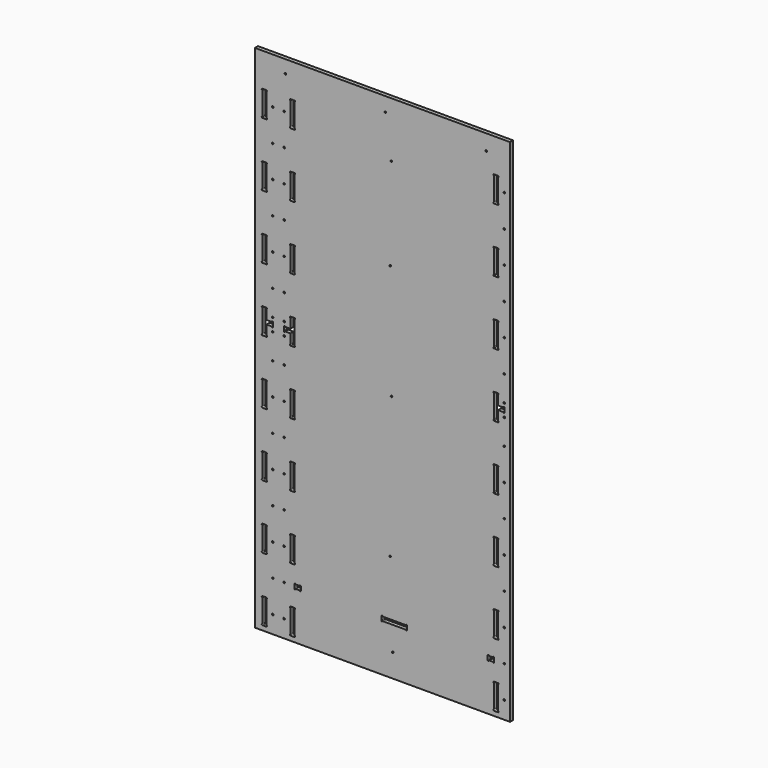
from build123d import *

# Parameters (mm, degrees)
F1_DEPTH = 18


# Not quite as in the source:
# - ends of sketch curves that miss each other by under 0.0002 mm in the source are joined


with BuildPart() as f1:
    # F0 (on Front) → F1 (new body)
    with BuildSketch(Plane.XZ):
        with BuildLine():
            Line((-600, 1063.948034), (-600, -1200))
            Line((-600, -1200), (599.502035, -1200))
            Line((599.502035, -1200), (599.501201, 1063.948272))
            Line((599.501201, 1063.948272), (115.500376, 1063.948245))
            Line((115.500376, 1063.948245), (115.500377, 1053.806799))
            ThreePointArc((115.500377, 1053.806799), (112.3608555537, 1050.5395429438), (108.9803764701, 1053.5568130354))
            Line((108.9803764701, 1053.5568130354), (1.52026, 1053.557046))
            ThreePointArc((1.52026, 1053.557046), (-1.8598651837, 1050.5493557616), (-4.9997393501, 1053.807060001))
            Line((-4.9997393501, 1053.807060001), (-4.999744, 1063.948265))
            Line((-4.999744, 1063.948265), (-600, 1063.948034))
        make_face()
        with BuildLine():
            ThreePointArc((-545.999425, -1057.5382900374), (-542.7418065766, -1060.6737091966), (-545.7494230529, -1064.0496793132))
            Line((-545.7494230529, -1064.0496793132), (-545.749383, -1172.027071))
            ThreePointArc((-545.749383, -1172.027071), (-542.7407774718, -1175.4030773266), (-545.999381, -1178.5384609569))
            Line((-545.999381, -1178.5384609569), (-564.499399, -1178.538468))
            ThreePointArc((-564.499399, -1178.538468), (-567.7570174234, -1175.4030488034), (-564.7494009471, -1172.0270786868))
            Line((-564.7494009471, -1172.0270786868), (-564.749441, -1064.049687))
            ThreePointArc((-564.749441, -1064.049687), (-567.7580465282, -1060.6736806734), (-564.499443, -1057.5382970431))
            Line((-564.499443, -1057.5382970431), (-545.999425, -1057.5382900374))
        make_face(mode=Mode.SUBTRACT)
        with BuildLine():
            ThreePointArc((-516.000128, -1121.775336), (-518.6517784294, -1120.6769864294), (-519.750128, -1118.025336))
            ThreePointArc((-519.750128, -1118.025336), (-518.6517784294, -1115.3736855706), (-516.000128, -1114.275336))
            ThreePointArc((-516.000128, -1114.275336), (-513.3484775706, -1115.3736855706), (-512.250128, -1118.025336))
            ThreePointArc((-512.250128, -1118.025336), (-513.3484775706, -1120.6769864294), (-516.000128, -1121.775336))
        make_face(mode=Mode.SUBTRACT)
        with BuildLine():
            ThreePointArc((-462.491463, -1121.775336), (-465.1431134294, -1120.6769864294), (-466.241463, -1118.025336))
            ThreePointArc((-466.241463, -1118.025336), (-465.1431134294, -1115.3736855706), (-462.491463, -1114.275336))
            ThreePointArc((-462.491463, -1114.275336), (-459.8398125706, -1115.3736855706), (-458.741463, -1118.025336))
            ThreePointArc((-458.741463, -1118.025336), (-459.8398125706, -1120.6769864294), (-462.491463, -1121.775336))
        make_face(mode=Mode.SUBTRACT)
        with BuildLine():
            ThreePointArc((-516.000128, -971.775336), (-518.6517784294, -970.6769864294), (-519.750128, -968.025336))
            ThreePointArc((-519.750128, -968.025336), (-518.6517784294, -965.3736855706), (-516.000128, -964.275336))
            ThreePointArc((-516.000128, -964.275336), (-513.3484775706, -965.3736855706), (-512.250128, -968.025336))
            ThreePointArc((-512.250128, -968.025336), (-513.3484775706, -970.6769864294), (-516.000128, -971.775336))
        make_face(mode=Mode.SUBTRACT)
        with BuildLine():
            ThreePointArc((-462.491463, -971.775336), (-465.1431134294, -970.6769864294), (-466.241463, -968.025336))
            ThreePointArc((-466.241463, -968.025336), (-465.1431134294, -965.3736855706), (-462.491463, -964.275336))
            ThreePointArc((-462.491463, -964.275336), (-459.8398125706, -965.3736855706), (-458.741463, -968.025336))
            ThreePointArc((-458.741463, -968.025336), (-459.8398125706, -970.6769864294), (-462.491463, -971.775336))
        make_face(mode=Mode.SUBTRACT)
        with BuildLine():
            Line((-432.749269, -1172.02703), (-432.749309, -1064.049638))
            ThreePointArc((-432.749309, -1064.049638), (-435.7579145282, -1060.6736316734), (-432.499311, -1057.5382480431))
            Line((-432.499311, -1057.5382480431), (-413.999293, -1057.538241))
            ThreePointArc((-413.999293, -1057.538241), (-410.7416745766, -1060.6736601966), (-413.7492910529, -1064.0496303132))
            Line((-413.7492910529, -1064.0496303132), (-413.749251, -1172.027023))
            ThreePointArc((-413.749251, -1172.027023), (-410.7406454718, -1175.4030293266), (-413.999249, -1178.5384129569))
            Line((-413.999249, -1178.5384129569), (-432.499267, -1178.538419))
            ThreePointArc((-432.499267, -1178.538419), (-435.7568854219, -1175.4029998417), (-432.749269, -1172.02703))
        make_face(mode=Mode.SUBTRACT)
        with BuildLine():
            ThreePointArc((-414.7479649626, -958.781652), (-411.6125458034, -955.5240335766), (-408.2365756868, -958.5316500529))
            Line((-408.2365756868, -958.5316500529), (-390.259321, -958.531643))
            ThreePointArc((-390.259321, -958.531643), (-386.8833146734, -955.5230374718), (-383.7479310431, -958.781641))
            Line((-383.7479310431, -958.781641), (-383.747925, -977.284785))
            ThreePointArc((-383.747925, -977.284785), (-386.8833441966, -980.5424034234), (-390.2593143132, -977.5347869471))
            Line((-390.2593143132, -977.5347869471), (-408.236569, -977.534794))
            ThreePointArc((-408.236569, -977.534794), (-411.6125753266, -980.5433995282), (-414.7479589569, -977.284796))
            Line((-414.7479589569, -977.284796), (-414.7479649626, -958.781652))
        make_face(mode=Mode.SUBTRACT)
        with BuildLine():
            ThreePointArc((-545.999537, -757.5282880373), (-542.7419175958, -760.663706697), (-545.7495340529, -764.0396773132))
            Line((-545.7495340529, -764.0396773132), (-545.749495, -872.016866))
            ThreePointArc((-545.749495, -872.016866), (-542.7408894527, -875.3928718269), (-545.999492, -878.5282559571))
            Line((-545.999492, -878.5282559571), (-564.49951, -878.528262))
            ThreePointArc((-564.49951, -878.528262), (-567.7571294027, -875.3928433414), (-564.7495130237, -872.0168726927))
            Line((-564.7495130237, -872.0168726927), (-564.749552, -764.039685))
            ThreePointArc((-564.749552, -764.039685), (-567.7581575473, -760.6636791731), (-564.499555, -757.5282950429))
            Line((-564.499555, -757.5282950429), (-545.999537, -757.5282880373))
        make_face(mode=Mode.SUBTRACT)
        with BuildLine():
            ThreePointArc((-516.000128, -821.775336), (-518.6517784294, -820.6769864294), (-519.750128, -818.025336))
            ThreePointArc((-519.750128, -818.025336), (-518.6517784294, -815.3736855706), (-516.000128, -814.275336))
            ThreePointArc((-516.000128, -814.275336), (-513.3484775706, -815.3736855706), (-512.250128, -818.025336))
            ThreePointArc((-512.250128, -818.025336), (-513.3484775706, -820.6769864294), (-516.000128, -821.775336))
        make_face(mode=Mode.SUBTRACT)
        with BuildLine():
            ThreePointArc((-462.491463, -821.775336), (-465.1431134294, -820.6769864294), (-466.241463, -818.025336))
            ThreePointArc((-466.241463, -818.025336), (-465.1431134294, -815.3736855706), (-462.491463, -814.275336))
            ThreePointArc((-462.491463, -814.275336), (-459.8398125706, -815.3736855706), (-458.741463, -818.025336))
            ThreePointArc((-458.741463, -818.025336), (-459.8398125706, -820.6769864294), (-462.491463, -821.775336))
        make_face(mode=Mode.SUBTRACT)
        with BuildLine():
            ThreePointArc((-516.000128, -671.775336), (-518.6517784294, -670.6769864294), (-519.750128, -668.025336))
            ThreePointArc((-519.750128, -668.025336), (-518.6517784294, -665.3736855706), (-516.000128, -664.275336))
            ThreePointArc((-516.000128, -664.275336), (-513.3484775706, -665.3736855706), (-512.250128, -668.025336))
            ThreePointArc((-512.250128, -668.025336), (-513.3484775706, -670.6769864294), (-516.000128, -671.775336))
        make_face(mode=Mode.SUBTRACT)
        with BuildLine():
            ThreePointArc((-462.491463, -671.775336), (-465.1431134294, -670.6769864294), (-466.241463, -668.025336))
            ThreePointArc((-466.241463, -668.025336), (-465.1431134294, -665.3736855706), (-462.491463, -664.275336))
            ThreePointArc((-462.491463, -664.275336), (-459.8398125706, -665.3736855706), (-458.741463, -668.025336))
            ThreePointArc((-458.741463, -668.025336), (-459.8398125706, -670.6769864294), (-462.491463, -671.775336))
        make_face(mode=Mode.SUBTRACT)
        with BuildLine():
            ThreePointArc((-432.7494189421, -764.0396352449), (-435.7580235481, -760.6636302113), (-432.499422, -757.5282470429))
            Line((-432.499422, -757.5282470429), (-413.999404, -757.52824))
            ThreePointArc((-413.999404, -757.52824), (-410.7417845973, -760.6636586586), (-413.7494009763, -764.0396293073))
            Line((-413.7494009763, -764.0396293073), (-413.749363, -872.016817))
            ThreePointArc((-413.749363, -872.016817), (-410.7407574527, -875.3928228269), (-413.99936, -878.5282069571))
            Line((-413.99936, -878.5282069571), (-432.499377, -878.528214))
            ThreePointArc((-432.499377, -878.528214), (-435.7569964042, -875.392795303), (-432.7493799471, -872.0168246868))
            Line((-432.7493799471, -872.0168246868), (-432.7494189421, -764.0396352449))
        make_face(mode=Mode.SUBTRACT)
        with BuildLine():
            ThreePointArc((-545.999646, -457.5277780374), (-542.7420275766, -460.6631971966), (-545.7496440529, -464.0391673132))
            Line((-545.7496440529, -464.0391673132), (-545.749604, -572.01656))
            ThreePointArc((-545.749604, -572.01656), (-542.7409984718, -575.3925663266), (-545.999602, -578.5279499569))
            Line((-545.999602, -578.5279499569), (-564.49962, -578.527957))
            ThreePointArc((-564.49962, -578.527957), (-567.7572384234, -575.3925378034), (-564.7496219471, -572.0165676868))
            Line((-564.7496219471, -572.0165676868), (-564.749662, -464.039175))
            ThreePointArc((-564.749662, -464.039175), (-567.7582675282, -460.6631686734), (-564.499664, -457.5277850431))
            Line((-564.499664, -457.5277850431), (-545.999646, -457.5277780374))
        make_face(mode=Mode.SUBTRACT)
        with BuildLine():
            ThreePointArc((-516.000128, -521.775336), (-518.6517784294, -520.6769864294), (-519.750128, -518.025336))
            ThreePointArc((-519.750128, -518.025336), (-518.6517784294, -515.3736855706), (-516.000128, -514.275336))
            ThreePointArc((-516.000128, -514.275336), (-513.3484775706, -515.3736855706), (-512.250128, -518.025336))
            ThreePointArc((-512.250128, -518.025336), (-513.3484775706, -520.6769864294), (-516.000128, -521.775336))
        make_face(mode=Mode.SUBTRACT)
        with BuildLine():
            ThreePointArc((-462.491463, -521.775336), (-465.1431134294, -520.6769864294), (-466.241463, -518.025336))
            ThreePointArc((-466.241463, -518.025336), (-465.1431134294, -515.3736855706), (-462.491463, -514.275336))
            ThreePointArc((-462.491463, -514.275336), (-459.8398125706, -515.3736855706), (-458.741463, -518.025336))
            ThreePointArc((-458.741463, -518.025336), (-459.8398125706, -520.6769864294), (-462.491463, -521.775336))
        make_face(mode=Mode.SUBTRACT)
        with BuildLine():
            ThreePointArc((-516.000128, -371.775336), (-518.6517784294, -370.6769864294), (-519.750128, -368.025336))
            ThreePointArc((-519.750128, -368.025336), (-518.6517784294, -365.3736855706), (-516.000128, -364.275336))
            ThreePointArc((-516.000128, -364.275336), (-513.3484775706, -365.3736855706), (-512.250128, -368.025336))
            ThreePointArc((-512.250128, -368.025336), (-513.3484775706, -370.6769864294), (-516.000128, -371.775336))
        make_face(mode=Mode.SUBTRACT)
        with BuildLine():
            ThreePointArc((-462.491463, -371.775336), (-465.1431134294, -370.6769864294), (-466.241463, -368.025336))
            ThreePointArc((-466.241463, -368.025336), (-465.1431134294, -365.3736855706), (-462.491463, -364.275336))
            ThreePointArc((-462.491463, -364.275336), (-459.8398125706, -365.3736855706), (-458.741463, -368.025336))
            ThreePointArc((-458.741463, -368.025336), (-459.8398125706, -370.6769864294), (-462.491463, -371.775336))
        make_face(mode=Mode.SUBTRACT)
        with BuildLine():
            ThreePointArc((-432.7495300186, -464.039126242), (-435.7581355282, -460.6631196734), (-432.499532, -457.5277360431))
            Line((-432.499532, -457.5277360431), (-413.999514, -457.52773))
            ThreePointArc((-413.999514, -457.52773), (-410.7418955781, -460.6631491583), (-413.7495119763, -464.0391193073))
            Line((-413.7495119763, -464.0391193073), (-413.749473, -572.016307))
            ThreePointArc((-413.749473, -572.016307), (-410.7408674718, -575.3923133266), (-413.999471, -578.5276969569))
            Line((-413.999471, -578.5276969569), (-432.499488, -578.527704))
            ThreePointArc((-432.499488, -578.527704), (-435.7571064234, -575.3922848034), (-432.7494899471, -572.0163146868))
            Line((-432.7494899471, -572.0163146868), (-432.7495300186, -464.039126242))
        make_face(mode=Mode.SUBTRACT)
        with BuildLine():
            ThreePointArc((-545.999757, -157.5272680374), (-542.7421385766, -160.6626871966), (-545.7497550529, -164.0386573132))
            Line((-545.7497550529, -164.0386573132), (-545.749715, -272.01605))
            ThreePointArc((-545.749715, -272.01605), (-542.7411094527, -275.3920558269), (-545.999712, -278.5274399571))
            Line((-545.999712, -278.5274399571), (-564.49973, -278.527446))
            ThreePointArc((-564.49973, -278.527446), (-567.7573494027, -275.3920273414), (-564.7497330237, -272.0160566927))
            Line((-564.7497330237, -272.0160566927), (-564.749773, -164.038665))
            ThreePointArc((-564.749773, -164.038665), (-567.7583785282, -160.6626586734), (-564.499775, -157.5272750431))
            Line((-564.499775, -157.5272750431), (-545.999757, -157.5272680374))
        make_face(mode=Mode.SUBTRACT)
        with BuildLine():
            ThreePointArc((-516.000128, -221.775336), (-518.6517784294, -220.6769864294), (-519.750128, -218.025336))
            ThreePointArc((-519.750128, -218.025336), (-518.6517784294, -215.3736855706), (-516.000128, -214.275336))
            ThreePointArc((-516.000128, -214.275336), (-513.3484775706, -215.3736855706), (-512.250128, -218.025336))
            ThreePointArc((-512.250128, -218.025336), (-513.3484775706, -220.6769864294), (-516.000128, -221.775336))
        make_face(mode=Mode.SUBTRACT)
        with BuildLine():
            ThreePointArc((-462.491463, -221.775336), (-465.1431134294, -220.6769864294), (-466.241463, -218.025336))
            ThreePointArc((-466.241463, -218.025336), (-465.1431134294, -215.3736855706), (-462.491463, -214.275336))
            ThreePointArc((-462.491463, -214.275336), (-459.8398125706, -215.3736855706), (-458.741463, -218.025336))
            ThreePointArc((-458.741463, -218.025336), (-459.8398125706, -220.6769864294), (-462.491463, -221.775336))
        make_face(mode=Mode.SUBTRACT)
        with BuildLine():
            ThreePointArc((-516.000128, -71.775336), (-518.6517784294, -70.6769864294), (-519.750128, -68.025336))
            ThreePointArc((-519.750128, -68.025336), (-518.6517784294, -65.3736855706), (-516.000128, -64.275336))
            ThreePointArc((-516.000128, -64.275336), (-513.3484775706, -65.3736855706), (-512.250128, -68.025336))
            ThreePointArc((-512.250128, -68.025336), (-513.3484775706, -70.6769864294), (-516.000128, -71.775336))
        make_face(mode=Mode.SUBTRACT)
        with BuildLine():
            ThreePointArc((-462.491463, -71.775336), (-465.1431134294, -70.6769864294), (-466.241463, -68.025336))
            ThreePointArc((-466.241463, -68.025336), (-465.1431134294, -65.3736855706), (-462.491463, -64.275336))
            ThreePointArc((-462.491463, -64.275336), (-459.8398125706, -65.3736855706), (-458.741463, -68.025336))
            ThreePointArc((-458.741463, -68.025336), (-459.8398125706, -70.6769864294), (-462.491463, -71.775336))
        make_face(mode=Mode.SUBTRACT)
        with BuildLine():
            ThreePointArc((-432.7496410186, -164.038616242), (-435.7582465282, -160.6626096734), (-432.499643, -157.5272260431))
            Line((-432.499643, -157.5272260431), (-413.999625, -157.527219))
            ThreePointArc((-413.999625, -157.527219), (-410.7420065766, -160.6626381966), (-413.7496230529, -164.0386083132))
            Line((-413.7496230529, -164.0386083132), (-413.749584, -272.015797))
            ThreePointArc((-413.749584, -272.015797), (-410.7409784527, -275.3918028269), (-413.999581, -278.5271869571))
            Line((-413.999581, -278.5271869571), (-432.499598, -278.527193))
            ThreePointArc((-432.499598, -278.527193), (-435.7572174027, -275.3917743414), (-432.7496010237, -272.0158036927))
            Line((-432.7496010237, -272.0158036927), (-432.7496410186, -164.038616242))
        make_face(mode=Mode.SUBTRACT)
        with BuildLine():
            ThreePointArc((44.445, -1090.918442), (45.5433495706, -1088.2667915706), (48.195, -1087.168442))
            ThreePointArc((48.195, -1087.168442), (50.8466504294, -1088.2667915706), (51.945, -1090.918442))
            ThreePointArc((51.945, -1090.918442), (50.8466504294, -1093.5700924294), (48.195, -1094.668442))
            ThreePointArc((48.195, -1094.668442), (45.5433495706, -1093.5700924294), (44.445, -1090.918442))
        make_face(mode=Mode.SUBTRACT)
        with BuildLine():
            ThreePointArc((1.263840242, -977.5348170186), (-2.1121658269, -980.5434225473), (-5.2475499571, -977.28482))
            Line((-5.2475499571, -977.28482), (-5.247556, -958.781327))
            ThreePointArc((-5.247556, -958.781327), (-2.1121368034, -955.5237085766), (1.2638333132, -958.5313250529))
            Line((1.2638333132, -958.5313250529), (109.241178, -958.531285))
            ThreePointArc((109.241178, -958.531285), (112.6171843266, -955.5226794718), (115.7525679569, -958.781283))
            Line((115.7525679569, -958.781283), (115.752574, -977.284775))
            ThreePointArc((115.752574, -977.284775), (112.6171548034, -980.5423934234), (109.2411846868, -977.5347769471))
            Line((109.2411846868, -977.5347769471), (1.263840242, -977.5348170186))
        make_face(mode=Mode.SUBTRACT)
        with BuildLine():
            ThreePointArc((32.71, -697.766442), (33.8083495706, -695.1147915706), (36.46, -694.016442))
            ThreePointArc((36.46, -694.016442), (39.1116504294, -695.1147915706), (40.21, -697.766442))
            ThreePointArc((40.21, -697.766442), (39.1116504294, -700.4180924294), (36.46, -701.516442))
            ThreePointArc((36.46, -701.516442), (33.8083495706, -700.4180924294), (32.71, -697.766442))
        make_face(mode=Mode.SUBTRACT)
        with BuildLine():
            ThreePointArc((524.2514499814, -1064.044670242), (521.2428444527, -1060.6686641731), (524.501447, -1057.5332800429))
            Line((524.501447, -1057.5332800429), (543.001465, -1057.533274))
            ThreePointArc((543.001465, -1057.533274), (546.2590844027, -1060.6686926586), (543.2514680237, -1064.0446633073))
            Line((543.2514680237, -1064.0446633073), (543.251507, -1172.022004))
            ThreePointArc((543.251507, -1172.022004), (546.2601125473, -1175.3980098269), (543.00151, -1178.5333939571))
            Line((543.00151, -1178.5333939571), (524.501492, -1178.5334))
            ThreePointArc((524.501492, -1178.5334), (521.2438725973, -1175.3979813414), (524.2514889763, -1172.0220106927))
            Line((524.2514889763, -1172.0220106927), (524.2514499814, -1064.044670242))
        make_face(mode=Mode.SUBTRACT)
        with BuildLine():
            ThreePointArc((572.885133, -1121.775336), (570.2334825706, -1120.6769864294), (569.135133, -1118.025336))
            ThreePointArc((569.135133, -1118.025336), (570.2334825706, -1115.3736855706), (572.885133, -1114.275336))
            ThreePointArc((572.885133, -1114.275336), (575.5367834294, -1115.3736855706), (576.635133, -1118.025336))
            ThreePointArc((576.635133, -1118.025336), (575.5367834294, -1120.6769864294), (572.885133, -1121.775336))
        make_face(mode=Mode.SUBTRACT)
        with BuildLine():
            ThreePointArc((500.7643391657, -977.5348480127), (497.3883316756, -980.5434524898), (494.2529490432, -977.284848))
            Line((494.2529490432, -977.284848), (494.252943, -958.78093))
            ThreePointArc((494.252943, -958.78093), (497.3883606992, -955.5233096341), (500.7643322366, -958.5309250588))
            Line((500.7643322366, -958.5309250588), (518.741583, -958.530911))
            ThreePointArc((518.741583, -958.530911), (522.1175878291, -955.5223044144), (525.2529729572, -958.780906))
            Line((525.2529729572, -958.780906), (525.252979, -977.28485))
            ThreePointArc((525.252979, -977.28485), (522.1175583074, -980.5424674808), (518.7415895336, -977.5348489589))
            Line((518.7415895336, -977.5348489589), (500.7643391657, -977.5348480127))
        make_face(mode=Mode.SUBTRACT)
        with BuildLine():
            ThreePointArc((572.885133, -971.775336), (570.2334825706, -970.6769864294), (569.135133, -968.025336))
            ThreePointArc((569.135133, -968.025336), (570.2334825706, -965.3736855706), (572.885133, -964.275336))
            ThreePointArc((572.885133, -964.275336), (575.5367834294, -965.3736855706), (576.635133, -968.025336))
            ThreePointArc((576.635133, -968.025336), (575.5367834294, -970.6769864294), (572.885133, -971.775336))
        make_face(mode=Mode.SUBTRACT)
        with BuildLine():
            ThreePointArc((543.2513960186, -872.021078758), (546.2600015282, -875.3970853266), (543.001398, -878.5324689569))
            Line((543.001398, -878.5324689569), (524.501381, -878.532476))
            ThreePointArc((524.501381, -878.532476), (521.2437625766, -875.3970568034), (524.2513790529, -872.0210866868))
            Line((524.2513790529, -872.0210866868), (524.251338, -764.04395))
            ThreePointArc((524.251338, -764.04395), (521.2427324527, -760.6679441731), (524.501335, -757.5325600429))
            Line((524.501335, -757.5325600429), (543.001353, -757.532553))
            ThreePointArc((543.001353, -757.532553), (546.2589724042, -760.667971697), (543.2513559471, -764.0439423132))
            Line((543.2513559471, -764.0439423132), (543.2513960186, -872.021078758))
        make_face(mode=Mode.SUBTRACT)
        with BuildLine():
            ThreePointArc((572.885133, -821.775336), (570.2334825706, -820.6769864294), (569.135133, -818.025336))
            ThreePointArc((569.135133, -818.025336), (570.2334825706, -815.3736855706), (572.885133, -814.275336))
            ThreePointArc((572.885133, -814.275336), (575.5367834294, -815.3736855706), (576.635133, -818.025336))
            ThreePointArc((576.635133, -818.025336), (575.5367834294, -820.6769864294), (572.885133, -821.775336))
        make_face(mode=Mode.SUBTRACT)
        with BuildLine():
            ThreePointArc((572.885133, -671.775336), (570.2334825706, -670.6769864294), (569.135133, -668.025336))
            ThreePointArc((569.135133, -668.025336), (570.2334825706, -665.3736855706), (572.885133, -664.275336))
            ThreePointArc((572.885133, -664.275336), (575.5367834294, -665.3736855706), (576.635133, -668.025336))
            ThreePointArc((576.635133, -668.025336), (575.5367834294, -670.6769864294), (572.885133, -671.775336))
        make_face(mode=Mode.SUBTRACT)
        with BuildLine():
            ThreePointArc((38.577, -33.984585), (39.6753495706, -31.3329345706), (42.327, -30.234585))
            ThreePointArc((42.327, -30.234585), (44.9786504294, -31.3329345706), (46.077, -33.984585))
            ThreePointArc((46.077, -33.984585), (44.9786504294, -36.6362354294), (42.327, -37.734585))
            ThreePointArc((42.327, -37.734585), (39.6753495706, -36.6362354294), (38.577, -33.984585))
        make_face(mode=Mode.SUBTRACT)
        with BuildLine():
            ThreePointArc((524.501271, -578.5319659627), (521.2436515958, -575.396547303), (524.2512680529, -572.0205766868))
            Line((524.2512680529, -572.0205766868), (524.251227, -464.04344))
            ThreePointArc((524.251227, -464.04344), (521.2426214718, -460.6674336734), (524.501225, -457.5320500431))
            Line((524.501225, -457.5320500431), (543.001243, -457.532043))
            ThreePointArc((543.001243, -457.532043), (546.2588614234, -460.6674621966), (543.2512449471, -464.0434323132))
            Line((543.2512449471, -464.0434323132), (543.251285, -572.020569))
            ThreePointArc((543.251285, -572.020569), (546.2598905282, -575.3965753266), (543.001287, -578.5319589569))
            Line((543.001287, -578.5319589569), (524.501271, -578.5319659627))
        make_face(mode=Mode.SUBTRACT)
        with BuildLine():
            ThreePointArc((572.885133, -521.775336), (570.2334825706, -520.6769864294), (569.135133, -518.025336))
            ThreePointArc((569.135133, -518.025336), (570.2334825706, -515.3736855706), (572.885133, -514.275336))
            ThreePointArc((572.885133, -514.275336), (575.5367834294, -515.3736855706), (576.635133, -518.025336))
            ThreePointArc((576.635133, -518.025336), (575.5367834294, -520.6769864294), (572.885133, -521.775336))
        make_face(mode=Mode.SUBTRACT)
        with BuildLine():
            ThreePointArc((572.885133, -371.775336), (570.2334825706, -370.6769864294), (569.135133, -368.025336))
            ThreePointArc((569.135133, -368.025336), (570.2334825706, -365.3736855706), (572.885133, -364.275336))
            ThreePointArc((572.885133, -364.275336), (575.5367834294, -365.3736855706), (576.635133, -368.025336))
            ThreePointArc((576.635133, -368.025336), (575.5367834294, -370.6769864294), (572.885133, -371.775336))
        make_face(mode=Mode.SUBTRACT)
        with BuildLine():
            ThreePointArc((543.2511740186, -272.020058758), (546.2597795473, -275.3960648269), (543.001177, -278.5314489571))
            Line((543.001177, -278.5314489571), (524.50116, -278.531455))
            ThreePointArc((524.50116, -278.531455), (521.2435415781, -275.3960358417), (524.2511579763, -272.0200656927))
            Line((524.2511579763, -272.0200656927), (524.251117, -164.04293))
            ThreePointArc((524.251117, -164.04293), (521.2425114527, -160.6669241731), (524.501114, -157.5315400429))
            Line((524.501114, -157.5315400429), (543.001132, -157.531533))
            ThreePointArc((543.001132, -157.531533), (546.2587514042, -160.666951697), (543.2511349471, -164.0429223132))
            Line((543.2511349471, -164.0429223132), (543.2511740186, -272.020058758))
        make_face(mode=Mode.SUBTRACT)
        with BuildLine():
            ThreePointArc((572.885133, -221.775336), (570.2334825706, -220.6769864294), (569.135133, -218.025336))
            ThreePointArc((569.135133, -218.025336), (570.2334825706, -215.3736855706), (572.885133, -214.275336))
            ThreePointArc((572.885133, -214.275336), (575.5367834294, -215.3736855706), (576.635133, -218.025336))
            ThreePointArc((576.635133, -218.025336), (575.5367834294, -220.6769864294), (572.885133, -221.775336))
        make_face(mode=Mode.SUBTRACT)
        with BuildLine():
            ThreePointArc((572.885133, -71.775336), (570.2334825706, -70.6769864294), (569.135133, -68.025336))
            ThreePointArc((569.135133, -68.025336), (570.2334825706, -65.3736855706), (572.885133, -64.275336))
            ThreePointArc((572.885133, -64.275336), (575.5367834294, -65.3736855706), (576.635133, -68.025336))
            ThreePointArc((576.635133, -68.025336), (575.5367834294, -70.6769864294), (572.885133, -71.775336))
        make_face(mode=Mode.SUBTRACT)
        with BuildLine():
            ThreePointArc((-545.999868, 142.4669129627), (-542.7422485958, 139.331494303), (-545.7498650529, 135.9555236868))
            Line((-545.7498650529, 135.9555236868), (-545.749849, 91.466836))
            Line((-545.749849, 91.466836), (-521.261208, 91.466846))
            ThreePointArc((-521.261208, 91.466846), (-517.8852016734, 94.4754515282), (-514.7498180431, 91.216848))
            Line((-514.7498180431, 91.216848), (-514.749811, 72.716827))
            ThreePointArc((-514.749811, 72.716827), (-517.8852521863, 69.4592297324), (-521.2612020042, 72.4668689997))
            Line((-521.2612020042, 72.4668689997), (-545.749843, 72.467028))
            Line((-545.749843, 72.467028), (-545.749827, 27.978336))
            ThreePointArc((-545.749827, 27.978336), (-542.7412214527, 24.6023301731), (-545.999824, 21.4669460429))
            Line((-545.999824, 21.4669460429), (-564.499841, 21.466939))
            ThreePointArc((-564.499841, 21.466939), (-567.7574594234, 24.6023581966), (-564.7498429471, 27.9783283132))
            Line((-564.7498429471, 27.9783283132), (-564.749884, 135.955516))
            ThreePointArc((-564.749884, 135.955516), (-567.7584895473, 139.3315218269), (-564.499887, 142.4669059571))
            Line((-564.499887, 142.4669059571), (-545.999868, 142.4669129627))
        make_face(mode=Mode.SUBTRACT)
        with BuildLine():
            ThreePointArc((-516.000128, 48.224664), (-518.6517784294, 49.3230135706), (-519.750128, 51.974664))
            ThreePointArc((-519.750128, 51.974664), (-518.6517784294, 54.6263144294), (-516.000128, 55.724664))
            ThreePointArc((-516.000128, 55.724664), (-513.3484775706, 54.6263144294), (-512.250128, 51.974664))
            ThreePointArc((-512.250128, 51.974664), (-513.3484775706, 49.3230135706), (-516.000128, 48.224664))
        make_face(mode=Mode.SUBTRACT)
        with BuildLine():
            ThreePointArc((-462.491463, 48.224664), (-465.1431134294, 49.3230135706), (-466.241463, 51.974664))
            ThreePointArc((-466.241463, 51.974664), (-465.1431134294, 54.6263144294), (-462.491463, 55.724664))
            ThreePointArc((-462.491463, 55.724664), (-459.8398125706, 54.6263144294), (-458.741463, 51.974664))
            ThreePointArc((-458.741463, 51.974664), (-459.8398125706, 49.3230135706), (-462.491463, 48.224664))
        make_face(mode=Mode.SUBTRACT)
        with BuildLine():
            ThreePointArc((-516.000128, 108.224664), (-518.6517784294, 109.3230135706), (-519.750128, 111.974664))
            ThreePointArc((-519.750128, 111.974664), (-518.6517784294, 114.6263144294), (-516.000128, 115.724664))
            ThreePointArc((-516.000128, 115.724664), (-513.3484775706, 114.6263144294), (-512.250128, 111.974664))
            ThreePointArc((-512.250128, 111.974664), (-513.3484775706, 109.3230135706), (-516.000128, 108.224664))
        make_face(mode=Mode.SUBTRACT)
        with BuildLine():
            ThreePointArc((-462.491463, 108.224664), (-465.1431134294, 109.3230135706), (-466.241463, 111.974664))
            ThreePointArc((-466.241463, 111.974664), (-465.1431134294, 114.6263144294), (-462.491463, 115.724664))
            ThreePointArc((-462.491463, 115.724664), (-459.8398125706, 114.6263144294), (-458.741463, 111.974664))
            ThreePointArc((-458.741463, 111.974664), (-459.8398125706, 109.3230135706), (-462.491463, 108.224664))
        make_face(mode=Mode.SUBTRACT)
        with BuildLine():
            ThreePointArc((-516.000128, 228.224664), (-518.6517784294, 229.3230135706), (-519.750128, 231.974664))
            ThreePointArc((-519.750128, 231.974664), (-518.6517784294, 234.6263144294), (-516.000128, 235.724664))
            ThreePointArc((-516.000128, 235.724664), (-513.3484775706, 234.6263144294), (-512.250128, 231.974664))
            ThreePointArc((-512.250128, 231.974664), (-513.3484775706, 229.3230135706), (-516.000128, 228.224664))
        make_face(mode=Mode.SUBTRACT)
        with BuildLine():
            ThreePointArc((-462.491463, 228.224664), (-465.1431134294, 229.3230135706), (-466.241463, 231.974664))
            ThreePointArc((-466.241463, 231.974664), (-465.1431134294, 234.6263144294), (-462.491463, 235.724664))
            ThreePointArc((-462.491463, 235.724664), (-459.8398125706, 234.6263144294), (-458.741463, 231.974664))
            ThreePointArc((-458.741463, 231.974664), (-459.8398125706, 229.3230135706), (-462.491463, 228.224664))
        make_face(mode=Mode.SUBTRACT)
        with BuildLine():
            ThreePointArc((-432.7497510186, 135.955564758), (-435.7583565473, 139.3315708269), (-432.499754, 142.4669549571))
            Line((-432.499754, 142.4669549571), (-413.999736, 142.466962))
            ThreePointArc((-413.999736, 142.466962), (-410.7421165958, 139.331543303), (-413.7497330529, 135.9555726868))
            Line((-413.7497330529, 135.9555726868), (-413.749694, 27.978385))
            ThreePointArc((-413.749694, 27.978385), (-410.7410884718, 24.6023786734), (-413.999692, 21.4669950431))
            Line((-413.999692, 21.4669950431), (-432.499709, 21.466988))
            ThreePointArc((-432.499709, 21.466988), (-435.7573274234, 24.6024071966), (-432.7497109471, 27.9783773132))
            Line((-432.7497109471, 27.9783773132), (-432.749728, 72.46686))
            Line((-432.749728, 72.46686), (-457.238369, 72.466851))
            ThreePointArc((-457.238369, 72.466851), (-460.6143753266, 69.4582454718), (-463.7497589569, 72.716849))
            Line((-463.7497589569, 72.716849), (-463.749766, 91.216864))
            ThreePointArc((-463.749766, 91.216864), (-460.6143688314, 94.4745035776), (-457.2383783839, 91.4669099704))
            Line((-457.2383783839, 91.4669099704), (-432.749736, 91.467088))
            Line((-432.749736, 91.467088), (-432.7497510186, 135.955564758))
        make_face(mode=Mode.SUBTRACT)
        with BuildLine():
            ThreePointArc((-545.999978, 442.4735929626), (-542.7423595766, 439.3381738034), (-545.7499760529, 435.9622036868))
            Line((-545.7499760529, 435.9622036868), (-545.749936, 327.984812))
            ThreePointArc((-545.749936, 327.984812), (-542.7413304718, 324.6088056734), (-545.999934, 321.4734220431))
            Line((-545.999934, 321.4734220431), (-564.499952, 321.473415))
            ThreePointArc((-564.499952, 321.473415), (-567.7575704234, 324.6088341966), (-564.7499539471, 327.9848043132))
            Line((-564.7499539471, 327.9848043132), (-564.749994, 435.962196))
            ThreePointArc((-564.749994, 435.962196), (-567.7585995282, 439.3382023266), (-564.499996, 442.4735859569))
            Line((-564.499996, 442.4735859569), (-545.999978, 442.4735929626))
        make_face(mode=Mode.SUBTRACT)
        with BuildLine():
            ThreePointArc((-516.000128, 378.224664), (-518.6517784294, 379.3230135706), (-519.750128, 381.974664))
            ThreePointArc((-519.750128, 381.974664), (-518.6517784294, 384.6263144294), (-516.000128, 385.724664))
            ThreePointArc((-516.000128, 385.724664), (-513.3484775706, 384.6263144294), (-512.250128, 381.974664))
            ThreePointArc((-512.250128, 381.974664), (-513.3484775706, 379.3230135706), (-516.000128, 378.224664))
        make_face(mode=Mode.SUBTRACT)
        with BuildLine():
            ThreePointArc((-462.491463, 378.224664), (-465.1431134294, 379.3230135706), (-466.241463, 381.974664))
            ThreePointArc((-466.241463, 381.974664), (-465.1431134294, 384.6263144294), (-462.491463, 385.724664))
            ThreePointArc((-462.491463, 385.724664), (-459.8398125706, 384.6263144294), (-458.741463, 381.974664))
            ThreePointArc((-458.741463, 381.974664), (-459.8398125706, 379.3230135706), (-462.491463, 378.224664))
        make_face(mode=Mode.SUBTRACT)
        with BuildLine():
            ThreePointArc((-516.000128, 528.224664), (-518.6517784294, 529.3230135706), (-519.750128, 531.974664))
            ThreePointArc((-519.750128, 531.974664), (-518.6517784294, 534.6263144294), (-516.000128, 535.724664))
            ThreePointArc((-516.000128, 535.724664), (-513.3484775706, 534.6263144294), (-512.250128, 531.974664))
            ThreePointArc((-512.250128, 531.974664), (-513.3484775706, 529.3230135706), (-516.000128, 528.224664))
        make_face(mode=Mode.SUBTRACT)
        with BuildLine():
            ThreePointArc((-462.491463, 528.224664), (-465.1431134294, 529.3230135706), (-466.241463, 531.974664))
            ThreePointArc((-466.241463, 531.974664), (-465.1431134294, 534.6263144294), (-462.491463, 535.724664))
            ThreePointArc((-462.491463, 535.724664), (-459.8398125706, 534.6263144294), (-458.741463, 531.974664))
            ThreePointArc((-458.741463, 531.974664), (-459.8398125706, 529.3230135706), (-462.491463, 528.224664))
        make_face(mode=Mode.SUBTRACT)
        with BuildLine():
            ThreePointArc((-432.7498620186, 435.962244758), (-435.7584675282, 439.3382513266), (-432.499864, 442.4736349569))
            Line((-432.499864, 442.4736349569), (-413.999846, 442.473642))
            ThreePointArc((-413.999846, 442.473642), (-410.7422275766, 439.3382228034), (-413.7498440529, 435.9622526868))
            Line((-413.7498440529, 435.9622526868), (-413.749805, 327.985065))
            ThreePointArc((-413.749805, 327.985065), (-410.7411994718, 324.6090586734), (-413.999803, 321.4736750431))
            Line((-413.999803, 321.4736750431), (-432.49982, 321.473668))
            ThreePointArc((-432.49982, 321.473668), (-435.7574384234, 324.6090871966), (-432.7498219471, 327.9850573132))
            Line((-432.7498219471, 327.9850573132), (-432.7498620186, 435.962244758))
        make_face(mode=Mode.SUBTRACT)
        Polygon((-32.274155, 136.734384), (-49.831488, 136.734384), (-49.831488, 156.705051), (-32.274155, 156.705051), (-31.779779, 156.701647), (-31.288275, 156.672696), (-30.800575, 156.61859), (-30.317613, 156.539717), (-29.840323, 156.43647), (-29.369639, 156.309238), (-28.906494, 156.158413), (-28.451821, 155.984384), (-28.006555, 155.787543), (-27.571629, 155.56828), (-27.147976, 155.326985), (-26.73653, 155.064051), (-26.338224, 154.779866), (-25.953993, 154.474821), (-25.58477, 154.149308), (-25.231488, 153.803717), (-24.891049, 153.452209), (-24.569978, 153.08528), (-24.26864, 152.703819), (-23.987405, 152.308717), (-23.726638, 151.900866), (-23.486707, 151.481155), (-23.267979, 151.050475), (-23.070821, 150.609717), (-22.895601, 150.159772), (-22.742686, 149.70153), (-22.612443, 149.235881), (-22.505238, 148.763717), (-22.42144, 148.285928), (-22.361415, 147.803405), (-22.325531, 147.317038), (-22.314155, 146.827717), (-22.311185, 146.326156), (-22.334025, 145.827103), (-22.382293, 145.331502), (-22.455613, 144.840301), (-22.553605, 144.354442), (-22.675889, 143.874873), (-22.822088, 143.402539), (-22.991821, 142.938384), (-23.184711, 142.483354), (-23.400379, 142.038394), (-23.638444, 141.60445), (-23.89853, 141.182467), (-24.180256, 140.77339), (-24.483243, 140.378165), (-24.807114, 139.997737), (-25.151488, 139.633051), (-25.511616, 139.288925), (-25.887384, 138.964795), (-26.277871, 138.661033), (-26.682155, 138.378009), (-27.099314, 138.116094), (-27.528426, 137.87566), (-27.968569, 137.657077), (-28.418821, 137.460717), (-28.878262, 137.286951), (-29.345967, 137.13615), (-29.821017, 137.008684), (-30.302488, 136.904926), (-30.789459, 136.825245), (-31.281009, 136.770014), (-31.776215, 136.739603), align=None, mode=Mode.SUBTRACT)
        with BuildLine():
            ThreePointArc((-546.000089, 742.4741029627), (-542.7424695973, 739.3386843414), (-545.7500859763, 735.9627136927))
            Line((-545.7500859763, 735.9627136927), (-545.750047, 627.985322))
            ThreePointArc((-545.750047, 627.985322), (-542.7414414527, 624.6093161731), (-546.000044, 621.4739320429))
            Line((-546.000044, 621.4739320429), (-564.500062, 621.473925))
            ThreePointArc((-564.500062, 621.473925), (-567.7576814042, 624.609343697), (-564.7500649471, 627.9853143132))
            Line((-564.7500649471, 627.9853143132), (-564.750104, 735.962707))
            ThreePointArc((-564.750104, 735.962707), (-567.7587085481, 739.3387127887), (-564.500107, 742.4740959571))
            Line((-564.500107, 742.4740959571), (-546.000089, 742.4741029627))
        make_face(mode=Mode.SUBTRACT)
        with BuildLine():
            ThreePointArc((-516.000128, 678.224664), (-518.6517784294, 679.3230135706), (-519.750128, 681.974664))
            ThreePointArc((-519.750128, 681.974664), (-518.6517784294, 684.6263144294), (-516.000128, 685.724664))
            ThreePointArc((-516.000128, 685.724664), (-513.3484775706, 684.6263144294), (-512.250128, 681.974664))
            ThreePointArc((-512.250128, 681.974664), (-513.3484775706, 679.3230135706), (-516.000128, 678.224664))
        make_face(mode=Mode.SUBTRACT)
        with BuildLine():
            ThreePointArc((-462.491463, 678.224664), (-465.1431134294, 679.3230135706), (-466.241463, 681.974664))
            ThreePointArc((-466.241463, 681.974664), (-465.1431134294, 684.6263144294), (-462.491463, 685.724664))
            ThreePointArc((-462.491463, 685.724664), (-459.8398125706, 684.6263144294), (-458.741463, 681.974664))
            ThreePointArc((-458.741463, 681.974664), (-459.8398125706, 679.3230135706), (-462.491463, 678.224664))
        make_face(mode=Mode.SUBTRACT)
        with BuildLine():
            ThreePointArc((-516.000128, 828.224664), (-518.6517784294, 829.3230135706), (-519.750128, 831.974664))
            ThreePointArc((-519.750128, 831.974664), (-518.6517784294, 834.6263144294), (-516.000128, 835.724664))
            ThreePointArc((-516.000128, 835.724664), (-513.3484775706, 834.6263144294), (-512.250128, 831.974664))
            ThreePointArc((-512.250128, 831.974664), (-513.3484775706, 829.3230135706), (-516.000128, 828.224664))
        make_face(mode=Mode.SUBTRACT)
        with BuildLine():
            ThreePointArc((-462.491463, 828.224664), (-465.1431134294, 829.3230135706), (-466.241463, 831.974664))
            ThreePointArc((-466.241463, 831.974664), (-465.1431134294, 834.6263144294), (-462.491463, 835.724664))
            ThreePointArc((-462.491463, 835.724664), (-459.8398125706, 834.6263144294), (-458.741463, 831.974664))
            ThreePointArc((-458.741463, 831.974664), (-459.8398125706, 829.3230135706), (-462.491463, 828.224664))
        make_face(mode=Mode.SUBTRACT)
        with BuildLine():
            ThreePointArc((-413.7499159814, 627.985575242), (-410.7413104527, 624.6095691731), (-413.999913, 621.4741850429))
            Line((-413.999913, 621.4741850429), (-432.49993, 621.474178))
            ThreePointArc((-432.49993, 621.474178), (-435.7575494042, 624.609596697), (-432.7499329471, 627.9855673132))
            Line((-432.7499329471, 627.9855673132), (-432.749972, 735.962755))
            ThreePointArc((-432.749972, 735.962755), (-435.7585775473, 739.3387608269), (-432.499975, 742.4741449571))
            Line((-432.499975, 742.4741449571), (-413.999957, 742.474152))
            ThreePointArc((-413.999957, 742.474152), (-410.7423385766, 739.3387328034), (-413.7499550529, 735.9627626868))
            Line((-413.7499550529, 735.9627626868), (-413.7499159814, 627.985575242))
        make_face(mode=Mode.SUBTRACT)
        with BuildLine():
            Line((-545.750198, 1035.962816), (-545.750158, 927.985629))
            ThreePointArc((-545.750158, 927.985629), (-542.7415524718, 924.6096226734), (-546.000156, 921.4742390431))
            Line((-546.000156, 921.4742390431), (-564.500174, 921.474232))
            ThreePointArc((-564.500174, 921.474232), (-567.7577924234, 924.6096511966), (-564.7501759471, 927.9856213132))
            Line((-564.7501759471, 927.9856213132), (-564.750216, 1035.962809))
            ThreePointArc((-564.750216, 1035.962809), (-567.7588215473, 1039.3388148269), (-564.500219, 1042.4741989571))
            Line((-564.500219, 1042.4741989571), (-546.000201, 1042.474206))
            ThreePointArc((-546.000201, 1042.474206), (-542.7425815958, 1039.338787303), (-545.750198, 1035.962816))
        make_face(mode=Mode.SUBTRACT)
        with BuildLine():
            ThreePointArc((-516.000128, 978.224664), (-518.6517784294, 979.3230135706), (-519.750128, 981.974664))
            ThreePointArc((-519.750128, 981.974664), (-518.6517784294, 984.6263144294), (-516.000128, 985.724664))
            ThreePointArc((-516.000128, 985.724664), (-513.3484775706, 984.6263144294), (-512.250128, 981.974664))
            ThreePointArc((-512.250128, 981.974664), (-513.3484775706, 979.3230135706), (-516.000128, 978.224664))
        make_face(mode=Mode.SUBTRACT)
        with BuildLine():
            ThreePointArc((-462.491463, 978.224664), (-465.1431134294, 979.3230135706), (-466.241463, 981.974664))
            ThreePointArc((-466.241463, 981.974664), (-465.1431134294, 984.6263144294), (-462.491463, 985.724664))
            ThreePointArc((-462.491463, 985.724664), (-459.8398125706, 984.6263144294), (-458.741463, 981.974664))
            ThreePointArc((-458.741463, 981.974664), (-459.8398125706, 979.3230135706), (-462.491463, 978.224664))
        make_face(mode=Mode.SUBTRACT)
        with BuildLine():
            ThreePointArc((-413.7500249814, 927.985473242), (-410.7414194718, 924.6094666734), (-414.000023, 921.4740830431))
            Line((-414.000023, 921.4740830431), (-432.500041, 921.474076))
            ThreePointArc((-432.500041, 921.474076), (-435.7576594234, 924.6094951966), (-432.7500429471, 927.9854653132))
            Line((-432.7500429471, 927.9854653132), (-432.750084, 1035.962858))
            ThreePointArc((-432.750084, 1035.962858), (-435.7586895473, 1039.3388638269), (-432.500087, 1042.4742479571))
            Line((-432.500087, 1042.4742479571), (-414.000067, 1042.474255))
            ThreePointArc((-414.000067, 1042.474255), (-410.7424485766, 1039.3388358034), (-413.7500650529, 1035.9628656868))
            Line((-413.7500650529, 1035.9628656868), (-413.7500249814, 927.985473242))
        make_face(mode=Mode.SUBTRACT)
        Polygon((3.387634, 116.187819), (2.973845, 116.185051), (2.553979, 116.181647), (2.135009, 116.188887), (1.717127, 116.206694), (1.300528, 116.234993), (0.885402, 116.273708), (0.471945, 116.322763), (0.060348, 116.382083), (-0.349196, 116.451592), (-0.756494, 116.531214), (-1.161353, 116.620874), (-1.56358, 116.720496), (-1.962983, 116.830004), (-2.359368, 116.949322), (-2.752542, 117.078375), (-3.142313, 117.217088), (-3.528488, 117.365384), (-3.910874, 117.523188), (-4.289278, 117.690424), (-4.663507, 117.867016), (-5.033368, 118.052889), (-5.398669, 118.247967), (-5.759217, 118.452175), (-6.114818, 118.665436), (-6.46528, 118.887676), (-6.81041, 119.118817), (-7.150015, 119.358786), (-7.483902, 119.607505), (-7.811879, 119.8649), (-8.133752, 120.130894), (-8.449329, 120.405412), (-8.758416, 120.688378), (-9.060821, 120.979717), (-9.410682, 121.359999), (-9.750203, 121.748187), (-10.079297, 122.144048), (-10.397874, 122.547347), (-10.705845, 122.957852), (-11.003122, 123.375329), (-11.289616, 123.799542), (-11.565238, 124.230259), (-11.829899, 124.667245), (-12.08351, 125.110267), (-12.325983, 125.559091), (-12.557228, 126.013483), (-12.777156, 126.473209), (-12.98568, 126.938034), (-13.182709, 127.407726), (-13.368155, 127.882051), (-13.541929, 128.360773), (-13.703943, 128.843661), (-13.854106, 129.330479), (-13.992332, 129.820993), (-14.11853, 130.314971), (-14.232612, 130.812178), (-14.334489, 131.312379), (-14.424071, 131.815342), (-14.501271, 132.320833), (-14.566, 132.828616), (-14.618168, 133.33846), (-14.657686, 133.850129), (-14.684466, 134.36339), (-14.698419, 134.878008), (-14.699456, 135.393751), (-14.687488, 135.910384), (-14.703559, 136.471505), (-14.705337, 137.031694), (-14.69292, 137.590694), (-14.666405, 138.148243), (-14.62589, 138.704084), (-14.571472, 139.257956), (-14.50325, 139.809601), (-14.421321, 140.358759), (-14.325783, 140.905171), (-14.216733, 141.448577), (-14.094269, 141.988719), (-13.958488, 142.525337), (-13.809489, 143.058172), (-13.647368, 143.586964), (-13.472224, 144.111454), (-13.284155, 144.631384), (-13.083257, 145.146493), (-12.869629, 145.656523), (-12.643368, 146.161213), (-12.404571, 146.660306), (-12.153338, 147.153541), (-11.889764, 147.640659), (-11.613948, 148.121402), (-11.325988, 148.595509), (-11.025981, 149.062722), (-10.714025, 149.52278), (-10.390217, 149.975426), (-10.054655, 150.4204), (-9.707437, 150.857441), (-9.34866, 151.286292), (-8.978422, 151.706693), (-8.596821, 152.118384), (-8.311073, 152.409058), (-8.018457, 152.691525), (-7.719171, 152.965704), (-7.41341, 153.231514), (-7.101369, 153.488873), (-6.783245, 153.737698), (-6.459233, 153.97791), (-6.12953, 154.209426), (-5.79433, 154.432164), (-5.45383, 154.646043), (-5.108225, 154.850982), (-4.757712, 155.0469), (-4.402486, 155.233713), (-4.042743, 155.411342), (-3.678678, 155.579703), (-3.310488, 155.738717), (-2.938368, 155.888301), (-2.562515, 156.028374), (-2.183123, 156.158854), (-1.800389, 156.27966), (-1.414509, 156.39071), (-1.025678, 156.491922), (-0.634092, 156.583216), (-0.239946, 156.664509), (0.156562, 156.73572), (0.555238, 156.796767), (0.955885, 156.84757), (1.358309, 156.888045), (1.762312, 156.918113), (2.1677, 156.937691), (2.574276, 156.946697), (2.981845, 156.945051), (3.396093, 156.941377), (3.809206, 156.926913), (4.220984, 156.901743), (4.631231, 156.865952), (5.039746, 156.819623), (5.446334, 156.762842), (5.850794, 156.695692), (6.252929, 156.618259), (6.65254, 156.530626), (7.04943, 156.432879), (7.4434, 156.325102), (7.834251, 156.207379), (8.221787, 156.079794), (8.605807, 155.942433), (8.986115, 155.795379), (9.362512, 155.638717), (9.734799, 155.472532), (10.102779, 155.296908), (10.466253, 155.111929), (10.825022, 154.917681), (11.17889, 154.714247), (11.527656, 154.501711), (11.871124, 154.28016), (12.209095, 154.049676), (12.541371, 153.810344), (12.867753, 153.562249), (13.188043, 153.305476), (13.502043, 153.040108), (13.809555, 152.76623), (14.11038, 152.483928), (14.404321, 152.193284), (14.691179, 151.894384), (15.061359, 151.484856), (15.420337, 151.066941), (15.768023, 150.640891), (16.104324, 150.206962), (16.429149, 149.765406), (16.742405, 149.316476), (17.044001, 148.860426), (17.333845, 148.397509), (17.611846, 147.927979), (17.87791, 147.452089), (18.131948, 146.970093), (18.373866, 146.482243), (18.603573, 145.988794), (18.820978, 145.489999), (19.025988, 144.986111), (19.218512, 144.477384), (19.398458, 143.964071), (19.565733, 143.446425), (19.720247, 142.9247), (19.861908, 142.39915), (19.990623, 141.870027), (20.106301, 141.337585), (20.20885, 140.802078), (20.298179, 140.263759), (20.374195, 139.722881), (20.436806, 139.179698), (20.485922, 138.634464), (20.521449, 138.087431), (20.543297, 137.538853), (20.551374, 136.988984), (20.545587, 136.438076), (20.525845, 135.886384), (20.534275, 135.371556), (20.529624, 134.857731), (20.511985, 134.345145), (20.481449, 133.834035), (20.438109, 133.324638), (20.382056, 132.817191), (20.313382, 132.31193), (20.232179, 131.809092), (20.138538, 131.308915), (20.032551, 130.811635), (19.91431, 130.317488), (19.783908, 129.826712), (19.641435, 129.339543), (19.486983, 128.856219), (19.320645, 128.376976), (19.142512, 127.902051), (18.952676, 127.43168), (18.751228, 126.966101), (18.538261, 126.50555), (18.313866, 126.050264), (18.078135, 125.60048), (17.83116, 125.156435), (17.573033, 124.718366), (17.303845, 124.286509), (17.023689, 123.861101), (16.732655, 123.442379), (16.430836, 123.03058), (16.118324, 122.625941), (15.795211, 122.228698), (15.461587, 121.839089), (15.117546, 121.45735), (14.763179, 121.083717), (14.469272, 120.792504), (14.168679, 120.509416), (13.861587, 120.234532), (13.548184, 119.967931), (13.228657, 119.709691), (12.903196, 119.459891), (12.571988, 119.21861), (12.23522, 118.985926), (11.893082, 118.761917), (11.54576, 118.546663), (11.193443, 118.340242), (10.836319, 118.142733), (10.474576, 117.954214), (10.108402, 117.774763), (9.737984, 117.604461), (9.363512, 117.443384), (8.985172, 117.291612), (8.603153, 117.149223), (8.217643, 117.016296), (7.82883, 116.89291), (7.436901, 116.779143), (7.042045, 116.675073), (6.64445, 116.58078), (6.244304, 116.496342), (5.841794, 116.421838), (5.437109, 116.357345), (5.030437, 116.302944), (4.621965, 116.258712), (4.211882, 116.224728), (3.800376, 116.201071), align=None, mode=Mode.SUBTRACT)
        Polygon((47.632968, 116.187819), (47.219179, 116.185051), (46.799312, 116.181647), (46.380342, 116.188887), (45.962461, 116.206694), (45.545861, 116.234993), (45.130736, 116.273708), (44.717278, 116.322763), (44.305681, 116.382083), (43.896137, 116.451592), (43.488839, 116.531214), (43.08398, 116.620874), (42.681753, 116.720496), (42.28235, 116.830004), (41.885966, 116.949322), (41.492791, 117.078375), (41.10302, 117.217088), (40.716845, 117.365384), (40.334459, 117.523188), (39.956056, 117.690424), (39.581826, 117.867016), (39.211965, 118.052889), (38.846664, 118.247967), (38.486117, 118.452175), (38.130516, 118.665436), (37.780054, 118.887676), (37.434924, 119.118817), (37.095319, 119.358786), (36.761431, 119.607505), (36.433455, 119.8649), (36.111581, 120.130894), (35.796005, 120.405412), (35.486917, 120.688378), (35.184512, 120.979717), (34.834652, 121.359999), (34.49513, 121.748187), (34.166037, 122.144048), (33.84746, 122.547347), (33.539488, 122.957852), (33.242211, 123.375329), (32.955717, 123.799542), (32.680095, 124.230259), (32.415434, 124.667245), (32.161823, 125.110267), (31.919351, 125.559091), (31.688106, 126.013483), (31.468177, 126.473209), (31.259654, 126.938034), (31.062625, 127.407726), (30.877179, 127.882051), (30.703404, 128.360773), (30.541391, 128.843661), (30.391227, 129.330479), (30.253001, 129.820993), (30.126803, 130.314971), (30.012722, 130.812178), (29.910845, 131.312379), (29.821262, 131.815342), (29.744062, 132.320833), (29.679334, 132.828616), (29.627166, 133.33846), (29.587647, 133.850129), (29.560867, 134.36339), (29.546914, 134.878008), (29.545877, 135.393751), (29.557845, 135.910384), (29.541774, 136.471505), (29.539996, 137.031694), (29.552414, 137.590694), (29.578929, 138.148243), (29.619444, 138.704084), (29.673861, 139.257956), (29.742083, 139.809601), (29.824012, 140.358759), (29.91955, 140.905171), (30.0286, 141.448577), (30.151065, 141.988719), (30.286845, 142.525337), (30.435845, 143.058172), (30.597965, 143.586964), (30.773109, 144.111454), (30.961179, 144.631384), (31.162076, 145.146493), (31.375705, 145.656523), (31.601966, 146.161213), (31.840762, 146.660306), (32.091996, 147.153541), (32.355569, 147.640659), (32.631385, 148.121402), (32.919345, 148.595509), (33.219352, 149.062722), (33.531309, 149.52278), (33.855117, 149.975426), (34.190679, 150.4204), (34.537897, 150.857441), (34.896673, 151.286292), (35.266911, 151.706693), (35.648512, 152.118384), (35.934261, 152.409058), (36.226876, 152.691525), (36.526162, 152.965704), (36.831923, 153.231514), (37.143964, 153.488873), (37.462088, 153.737698), (37.7861, 153.97791), (38.115804, 154.209426), (38.451003, 154.432164), (38.791503, 154.646043), (39.137108, 154.850982), (39.487621, 155.0469), (39.842847, 155.233713), (40.202591, 155.411342), (40.566655, 155.579703), (40.934845, 155.738717), (41.306965, 155.888301), (41.682819, 156.028374), (42.06221, 156.158854), (42.444944, 156.27966), (42.830825, 156.39071), (43.219656, 156.491922), (43.611242, 156.583216), (44.005387, 156.664509), (44.401895, 156.73572), (44.800571, 156.796767), (45.201219, 156.84757), (45.603642, 156.888045), (46.007646, 156.918113), (46.413033, 156.937691), (46.81961, 156.946697), (47.227179, 156.945051), (47.641427, 156.941377), (48.054539, 156.926913), (48.466318, 156.901743), (48.876564, 156.865952), (49.28508, 156.819623), (49.691667, 156.762842), (50.096127, 156.695692), (50.498262, 156.618259), (50.897873, 156.530626), (51.294763, 156.432879), (51.688733, 156.325102), (52.079585, 156.207379), (52.46712, 156.079794), (52.851141, 155.942433), (53.231449, 155.795379), (53.607845, 155.638717), (53.980133, 155.472532), (54.348112, 155.296908), (54.711586, 155.111929), (55.070356, 154.917681), (55.424223, 154.714247), (55.77299, 154.501711), (56.116458, 154.28016), (56.454429, 154.049676), (56.786704, 153.810344), (57.113086, 153.562249), (57.433376, 153.305476), (57.747376, 153.040108), (58.054888, 152.76623), (58.355714, 152.483928), (58.649654, 152.193284), (58.936512, 151.894384), (59.306692, 151.484856), (59.665671, 151.066941), (60.013357, 150.640891), (60.349658, 150.206962), (60.674482, 149.765406), (60.987738, 149.316476), (61.289334, 148.860426), (61.579179, 148.397509), (61.857179, 147.927979), (62.123244, 147.452089), (62.377281, 146.970093), (62.619199, 146.482243), (62.848907, 145.988794), (63.066311, 145.489999), (63.271321, 144.986111), (63.463845, 144.477384), (63.643791, 143.964071), (63.811067, 143.446425), (63.965581, 142.9247), (64.107241, 142.39915), (64.235956, 141.870027), (64.351634, 141.337585), (64.454183, 140.802078), (64.543512, 140.263759), (64.619528, 139.722881), (64.68214, 139.179698), (64.731255, 138.634464), (64.766783, 138.087431), (64.788631, 137.538853), (64.796707, 136.988984), (64.79092, 136.438076), (64.771179, 135.886384), (64.779608, 135.371556), (64.774957, 134.857731), (64.757318, 134.345145), (64.726783, 133.834035), (64.683443, 133.324638), (64.62739, 132.817191), (64.558715, 132.31193), (64.477512, 131.809092), (64.383871, 131.308915), (64.277884, 130.811635), (64.159644, 130.317488), (64.029241, 129.826712), (63.886768, 129.339543), (63.732317, 128.856219), (63.565978, 128.376976), (63.387845, 127.902051), (63.198009, 127.43168), (62.996561, 126.966101), (62.783594, 126.50555), (62.559199, 126.050264), (62.323469, 125.60048), (62.076494, 125.156435), (61.818366, 124.718366), (61.549179, 124.286509), (61.269022, 123.861101), (60.977988, 123.442379), (60.67617, 123.03058), (60.363658, 122.625941), (60.040544, 122.228698), (59.706921, 121.839089), (59.362879, 121.45735), (59.008512, 121.083717), (58.714606, 120.792504), (58.414013, 120.509416), (58.10692, 120.234532), (57.793517, 119.967931), (57.473991, 119.709691), (57.148529, 119.459891), (56.817321, 119.21861), (56.480554, 118.985926), (56.138415, 118.761917), (55.791093, 118.546663), (55.438776, 118.340242), (55.081653, 118.142733), (54.719909, 117.954214), (54.353735, 117.774763), (53.983318, 117.604461), (53.608845, 117.443384), (53.230505, 117.291612), (52.848487, 117.149223), (52.462976, 117.016296), (52.074163, 116.89291), (51.682234, 116.779143), (51.287378, 116.675073), (50.889783, 116.58078), (50.489637, 116.496342), (50.087127, 116.421838), (49.682442, 116.357345), (49.27577, 116.302944), (48.867298, 116.258712), (48.457215, 116.224728), (48.045709, 116.201071), align=None, mode=Mode.SUBTRACT)
        with BuildLine():
            ThreePointArc((32.71, 505.161558), (33.8083495706, 507.8132084294), (36.46, 508.911558))
            ThreePointArc((36.46, 508.911558), (39.1116504294, 507.8132084294), (40.21, 505.161558))
            ThreePointArc((40.21, 505.161558), (39.1116504294, 502.5099075706), (36.46, 501.411558))
            ThreePointArc((36.46, 501.411558), (33.8083495706, 502.5099075706), (32.71, 505.161558))
        make_face(mode=Mode.SUBTRACT)
        with BuildLine():
            ThreePointArc((572.885133, 48.224664), (570.2334825706, 49.3230135706), (569.135133, 51.974664))
            ThreePointArc((569.135133, 51.974664), (570.2334825706, 54.6263144294), (572.885133, 55.724664))
            ThreePointArc((572.885133, 55.724664), (575.5367834294, 54.6263144294), (576.635133, 51.974664))
            ThreePointArc((576.635133, 51.974664), (575.5367834294, 49.3230135706), (572.885133, 48.224664))
        make_face(mode=Mode.SUBTRACT)
        with BuildLine():
            ThreePointArc((524.501049, 21.4690550374), (521.2434305766, 24.6044741966), (524.2510470529, 27.9804443132))
            Line((524.2510470529, 27.9804443132), (524.251006, 135.957581))
            ThreePointArc((524.251006, 135.957581), (521.2424004718, 139.3335873266), (524.501004, 142.4689709569))
            Line((524.501004, 142.4689709569), (543.001023, 142.468977))
            ThreePointArc((543.001023, 142.468977), (546.2586414219, 139.3335578417), (543.2510250237, 135.9575876927))
            Line((543.2510250237, 135.9575876927), (543.251041, 91.468927))
            Line((543.251041, 91.468927), (567.739683, 91.468936))
            ThreePointArc((567.739683, 91.468936), (571.1156893266, 94.4775415282), (574.2510729569, 91.218938))
            Line((574.2510729569, 91.218938), (574.251079, 72.718917))
            ThreePointArc((574.251079, 72.718917), (571.1156378137, 69.4613197324), (567.7396879958, 72.4689589997))
            Line((567.7396879958, 72.4689589997), (543.251047, 72.469118))
            Line((543.251047, 72.469118), (543.251064, 27.980452))
            ThreePointArc((543.251064, 27.980452), (546.2596695282, 24.6044456734), (543.001066, 21.4690620431))
            Line((543.001066, 21.4690620431), (524.501049, 21.4690550374))
        make_face(mode=Mode.SUBTRACT)
        with BuildLine():
            ThreePointArc((572.885133, 108.224664), (570.2334825706, 109.3230135706), (569.135133, 111.974664))
            ThreePointArc((569.135133, 111.974664), (570.2334825706, 114.6263144294), (572.885133, 115.724664))
            ThreePointArc((572.885133, 115.724664), (575.5367834294, 114.6263144294), (576.635133, 111.974664))
            ThreePointArc((576.635133, 111.974664), (575.5367834294, 109.3230135706), (572.885133, 108.224664))
        make_face(mode=Mode.SUBTRACT)
        with BuildLine():
            ThreePointArc((572.885133, 228.224664), (570.2334825706, 229.3230135706), (569.135133, 231.974664))
            ThreePointArc((569.135133, 231.974664), (570.2334825706, 234.6263144294), (572.885133, 235.724664))
            ThreePointArc((572.885133, 235.724664), (575.5367834294, 234.6263144294), (576.635133, 231.974664))
            ThreePointArc((576.635133, 231.974664), (575.5367834294, 229.3230135706), (572.885133, 228.224664))
        make_face(mode=Mode.SUBTRACT)
        with BuildLine():
            ThreePointArc((524.500939, 321.4694060373), (521.2433195958, 324.604824697), (524.2509360529, 327.9807953132))
            Line((524.2509360529, 327.9807953132), (524.250896, 435.957932))
            ThreePointArc((524.250896, 435.957932), (521.2422904527, 439.3339378269), (524.500893, 442.4693219571))
            Line((524.500893, 442.4693219571), (543.000911, 442.469328))
            ThreePointArc((543.000911, 442.469328), (546.2585294219, 439.3339088417), (543.2509130237, 435.9579386927))
            Line((543.2509130237, 435.9579386927), (543.250953, 327.980803))
            ThreePointArc((543.250953, 327.980803), (546.2595585473, 324.6047971731), (543.000956, 321.4694130429))
            Line((543.000956, 321.4694130429), (524.500939, 321.4694060373))
        make_face(mode=Mode.SUBTRACT)
        with BuildLine():
            ThreePointArc((572.885133, 378.224664), (570.2334825706, 379.3230135706), (569.135133, 381.974664))
            ThreePointArc((569.135133, 381.974664), (570.2334825706, 384.6263144294), (572.885133, 385.724664))
            ThreePointArc((572.885133, 385.724664), (575.5367834294, 384.6263144294), (576.635133, 381.974664))
            ThreePointArc((576.635133, 381.974664), (575.5367834294, 379.3230135706), (572.885133, 378.224664))
        make_face(mode=Mode.SUBTRACT)
        with BuildLine():
            ThreePointArc((572.885133, 528.224664), (570.2334825706, 529.3230135706), (569.135133, 531.974664))
            ThreePointArc((569.135133, 531.974664), (570.2334825706, 534.6263144294), (572.885133, 535.724664))
            ThreePointArc((572.885133, 535.724664), (575.5367834294, 534.6263144294), (576.635133, 531.974664))
            ThreePointArc((576.635133, 531.974664), (575.5367834294, 529.3230135706), (572.885133, 528.224664))
        make_face(mode=Mode.SUBTRACT)
        with BuildLine():
            ThreePointArc((38.577, 939.389558), (39.6753495706, 942.0412084294), (42.327, 943.139558))
            ThreePointArc((42.327, 943.139558), (44.9786504294, 942.0412084294), (46.077, 939.389558))
            ThreePointArc((46.077, 939.389558), (44.9786504294, 936.7379075706), (42.327, 935.639558))
            ThreePointArc((42.327, 935.639558), (39.6753495706, 936.7379075706), (38.577, 939.389558))
        make_face(mode=Mode.SUBTRACT)
        with BuildLine():
            ThreePointArc((524.500828, 621.4699160374), (521.2432095766, 624.6053351966), (524.2508260529, 627.9813053132))
            Line((524.2508260529, 627.9813053132), (524.250785, 735.958442))
            ThreePointArc((524.250785, 735.958442), (521.2421794527, 739.3344478269), (524.500782, 742.4698319571))
            Line((524.500782, 742.4698319571), (543.0008, 742.469839))
            ThreePointArc((543.0008, 742.469839), (546.2584194042, 739.334420303), (543.2508029471, 735.9584496868))
            Line((543.2508029471, 735.9584496868), (543.250843, 627.981313))
            ThreePointArc((543.250843, 627.981313), (546.2594485282, 624.6053066734), (543.000845, 621.4699230431))
            Line((543.000845, 621.4699230431), (524.500828, 621.4699160374))
        make_face(mode=Mode.SUBTRACT)
        with BuildLine():
            ThreePointArc((572.885133, 678.224664), (570.2334825706, 679.3230135706), (569.135133, 681.974664))
            ThreePointArc((569.135133, 681.974664), (570.2334825706, 684.6263144294), (572.885133, 685.724664))
            ThreePointArc((572.885133, 685.724664), (575.5367834294, 684.6263144294), (576.635133, 681.974664))
            ThreePointArc((576.635133, 681.974664), (575.5367834294, 679.3230135706), (572.885133, 678.224664))
        make_face(mode=Mode.SUBTRACT)
        with BuildLine():
            ThreePointArc((572.885133, 828.224664), (570.2334825706, 829.3230135706), (569.135133, 831.974664))
            ThreePointArc((569.135133, 831.974664), (570.2334825706, 834.6263144294), (572.885133, 835.724664))
            ThreePointArc((572.885133, 835.724664), (575.5367834294, 834.6263144294), (576.635133, 831.974664))
            ThreePointArc((576.635133, 831.974664), (575.5367834294, 829.3230135706), (572.885133, 828.224664))
        make_face(mode=Mode.SUBTRACT)
        with BuildLine():
            ThreePointArc((524.500718, 921.4704260373), (521.2430985958, 924.605844697), (524.2507150529, 927.9818153132))
            Line((524.2507150529, 927.9818153132), (524.250674, 1035.958952))
            ThreePointArc((524.250674, 1035.958952), (521.2420684718, 1039.3349583266), (524.500672, 1042.4703419569))
            Line((524.500672, 1042.4703419569), (543.00069, 1042.470349))
            ThreePointArc((543.00069, 1042.470349), (546.2583084234, 1039.3349298034), (543.2506919471, 1035.9589596868))
            Line((543.2506919471, 1035.9589596868), (543.250732, 927.981823))
            ThreePointArc((543.250732, 927.981823), (546.2593375282, 924.6058166734), (543.000734, 921.4704330431))
            Line((543.000734, 921.4704330431), (524.500718, 921.4704260373))
        make_face(mode=Mode.SUBTRACT)
        with BuildLine():
            ThreePointArc((572.885133, 978.224664), (570.2334825706, 979.3230135706), (569.135133, 981.974664))
            ThreePointArc((569.135133, 981.974664), (570.2334825706, 984.6263144294), (572.885133, 985.724664))
            ThreePointArc((572.885133, 985.724664), (575.5367834294, 984.6263144294), (576.635133, 981.974664))
            ThreePointArc((576.635133, 981.974664), (575.5367834294, 979.3230135706), (572.885133, 978.224664))
        make_face(mode=Mode.SUBTRACT)
        with BuildLine():
            Line((599.501201, 1063.948272), (599.502035, -1200))
            Line((599.502035, -1200), (600, -1200))
            Line((600, -1200), (600, 1200))
            Line((600, 1200), (-600, 1200))
            Line((-600, 1200), (-600, 1063.948034))
            Line((-600, 1063.948034), (-4.999744, 1063.948265))
            Line((-4.999744, 1063.948265), (-4.99974, 1053.80706))
            ThreePointArc((-4.99974, 1053.80706), (-1.8598651837, 1050.5493557616), (1.5202599785, 1053.5570460017))
            Line((1.5202599785, 1053.5570460017), (108.980376, 1053.556813))
            ThreePointArc((108.980376, 1053.556813), (112.3608555537, 1050.5395429438), (115.5003770941, 1053.8067990001))
            Line((115.5003770941, 1053.8067990001), (115.500376, 1063.948245))
            Line((115.500376, 1063.948245), (599.501201, 1063.948272))
        make_face()
        with BuildLine():
            ThreePointArc((-460.198, 1138.899558), (-459.0996504294, 1141.5512084294), (-456.448, 1142.649558))
            ThreePointArc((-456.448, 1142.649558), (-453.7963495706, 1141.5512084294), (-452.698, 1138.899558))
            ThreePointArc((-452.698, 1138.899558), (-453.7963495706, 1136.2479075706), (-456.448, 1135.149558))
            ThreePointArc((-456.448, 1135.149558), (-459.0996504294, 1136.2479075706), (-460.198, 1138.899558))
        make_face(mode=Mode.SUBTRACT)
        with BuildLine():
            ThreePointArc((9.238, 1133.031558), (10.3363495706, 1135.6832084294), (12.988, 1136.781558))
            ThreePointArc((12.988, 1136.781558), (15.6396504294, 1135.6832084294), (16.738, 1133.031558))
            ThreePointArc((16.738, 1133.031558), (15.6396504294, 1130.3799075706), (12.988, 1129.281558))
            ThreePointArc((12.988, 1129.281558), (10.3363495706, 1130.3799075706), (9.238, 1133.031558))
        make_face(mode=Mode.SUBTRACT)
        with BuildLine():
            ThreePointArc((484.541, 1127.163558), (485.6393495706, 1129.8152084294), (488.291, 1130.913558))
            ThreePointArc((488.291, 1130.913558), (490.9426504294, 1129.8152084294), (492.041, 1127.163558))
            ThreePointArc((492.041, 1127.163558), (490.9426504294, 1124.5119075706), (488.291, 1123.413558))
            ThreePointArc((488.291, 1123.413558), (485.6393495706, 1124.5119075706), (484.541, 1127.163558))
        make_face(mode=Mode.SUBTRACT)
        Polygon((-49.831488, 156.705051), (-49.831488, 136.734384), (-32.274155, 136.734384), (-31.776215, 136.739603), (-31.281009, 136.770014), (-30.789459, 136.825245), (-30.302488, 136.904926), (-29.821017, 137.008684), (-29.345967, 137.13615), (-28.878262, 137.286951), (-28.418821, 137.460717), (-27.968569, 137.657077), (-27.528426, 137.87566), (-27.099314, 138.116094), (-26.682155, 138.378009), (-26.277871, 138.661033), (-25.887384, 138.964795), (-25.511616, 139.288925), (-25.151488, 139.633051), (-24.807114, 139.997737), (-24.483243, 140.378165), (-24.180256, 140.77339), (-23.89853, 141.182467), (-23.638444, 141.60445), (-23.400379, 142.038394), (-23.184711, 142.483354), (-22.991821, 142.938384), (-22.822088, 143.402539), (-22.675889, 143.874873), (-22.553605, 144.354442), (-22.455613, 144.840301), (-22.382293, 145.331502), (-22.334025, 145.827103), (-22.311185, 146.326156), (-22.314155, 146.827717), (-22.325531, 147.317038), (-22.361415, 147.803405), (-22.42144, 148.285928), (-22.505238, 148.763717), (-22.612443, 149.235881), (-22.742686, 149.70153), (-22.895601, 150.159772), (-23.070821, 150.609717), (-23.267979, 151.050475), (-23.486707, 151.481155), (-23.726638, 151.900866), (-23.987405, 152.308717), (-24.26864, 152.703819), (-24.569978, 153.08528), (-24.891049, 153.452209), (-25.231488, 153.803717), (-25.58477, 154.149308), (-25.953993, 154.474821), (-26.338224, 154.779866), (-26.73653, 155.064051), (-27.147976, 155.326985), (-27.571629, 155.56828), (-28.006555, 155.787543), (-28.451821, 155.984384), (-28.906494, 156.158413), (-29.369639, 156.309238), (-29.840323, 156.43647), (-30.317613, 156.539717), (-30.800575, 156.61859), (-31.288275, 156.672696), (-31.779779, 156.701647), (-32.274155, 156.705051), align=None)
        Polygon((2.553979, 116.181647), (2.973845, 116.185051), (3.387634, 116.187819), (3.800376, 116.201071), (4.211882, 116.224728), (4.621965, 116.258712), (5.030437, 116.302944), (5.437109, 116.357345), (5.841794, 116.421838), (6.244304, 116.496342), (6.64445, 116.58078), (7.042045, 116.675073), (7.436901, 116.779143), (7.82883, 116.89291), (8.217643, 117.016296), (8.603153, 117.149223), (8.985172, 117.291612), (9.363512, 117.443384), (9.737984, 117.604461), (10.108402, 117.774763), (10.474576, 117.954214), (10.836319, 118.142733), (11.193443, 118.340242), (11.54576, 118.546663), (11.893082, 118.761917), (12.23522, 118.985926), (12.571988, 119.21861), (12.903196, 119.459891), (13.228657, 119.709691), (13.548184, 119.967931), (13.861587, 120.234532), (14.168679, 120.509416), (14.469272, 120.792504), (14.763179, 121.083717), (15.117546, 121.45735), (15.461587, 121.839089), (15.795211, 122.228698), (16.118324, 122.625941), (16.430836, 123.03058), (16.732655, 123.442379), (17.023689, 123.861101), (17.303845, 124.286509), (17.573033, 124.718366), (17.83116, 125.156435), (18.078135, 125.60048), (18.313866, 126.050264), (18.538261, 126.50555), (18.751228, 126.966101), (18.952676, 127.43168), (19.142512, 127.902051), (19.320645, 128.376976), (19.486983, 128.856219), (19.641435, 129.339543), (19.783908, 129.826712), (19.91431, 130.317488), (20.032551, 130.811635), (20.138538, 131.308915), (20.232179, 131.809092), (20.313382, 132.31193), (20.382056, 132.817191), (20.438109, 133.324638), (20.481449, 133.834035), (20.511985, 134.345145), (20.529624, 134.857731), (20.534275, 135.371556), (20.525845, 135.886384), (20.545587, 136.438076), (20.551374, 136.988984), (20.543297, 137.538853), (20.521449, 138.087431), (20.485922, 138.634464), (20.436806, 139.179698), (20.374195, 139.722881), (20.298179, 140.263759), (20.20885, 140.802078), (20.106301, 141.337585), (19.990623, 141.870027), (19.861908, 142.39915), (19.720247, 142.9247), (19.565733, 143.446425), (19.398458, 143.964071), (19.218512, 144.477384), (19.025988, 144.986111), (18.820978, 145.489999), (18.603573, 145.988794), (18.373866, 146.482243), (18.131948, 146.970093), (17.87791, 147.452089), (17.611846, 147.927979), (17.333845, 148.397509), (17.044001, 148.860426), (16.742405, 149.316476), (16.429149, 149.765406), (16.104324, 150.206962), (15.768023, 150.640891), (15.420337, 151.066941), (15.061359, 151.484856), (14.691179, 151.894384), (14.404321, 152.193284), (14.11038, 152.483928), (13.809555, 152.76623), (13.502043, 153.040108), (13.188043, 153.305476), (12.867753, 153.562249), (12.541371, 153.810344), (12.209095, 154.049676), (11.871124, 154.28016), (11.527656, 154.501711), (11.17889, 154.714247), (10.825022, 154.917681), (10.466253, 155.111929), (10.102779, 155.296908), (9.734799, 155.472532), (9.362512, 155.638717), (8.986115, 155.795379), (8.605807, 155.942433), (8.221787, 156.079794), (7.834251, 156.207379), (7.4434, 156.325102), (7.04943, 156.432879), (6.65254, 156.530626), (6.252929, 156.618259), (5.850794, 156.695692), (5.446334, 156.762842), (5.039746, 156.819623), (4.631231, 156.865952), (4.220984, 156.901743), (3.809206, 156.926913), (3.396093, 156.941377), (2.981845, 156.945051), (2.574276, 156.946697), (2.1677, 156.937691), (1.762312, 156.918113), (1.358309, 156.888045), (0.955885, 156.84757), (0.555238, 156.796767), (0.156562, 156.73572), (-0.239946, 156.664509), (-0.634092, 156.583216), (-1.025678, 156.491922), (-1.414509, 156.39071), (-1.800389, 156.27966), (-2.183123, 156.158854), (-2.562515, 156.028374), (-2.938368, 155.888301), (-3.310488, 155.738717), (-3.678678, 155.579703), (-4.042743, 155.411342), (-4.402486, 155.233713), (-4.757712, 155.0469), (-5.108225, 154.850982), (-5.45383, 154.646043), (-5.79433, 154.432164), (-6.12953, 154.209426), (-6.459233, 153.97791), (-6.783245, 153.737698), (-7.101369, 153.488873), (-7.41341, 153.231514), (-7.719171, 152.965704), (-8.018457, 152.691525), (-8.311073, 152.409058), (-8.596821, 152.118384), (-8.978422, 151.706693), (-9.34866, 151.286292), (-9.707437, 150.857441), (-10.054655, 150.4204), (-10.390217, 149.975426), (-10.714025, 149.52278), (-11.025981, 149.062722), (-11.325988, 148.595509), (-11.613948, 148.121402), (-11.889764, 147.640659), (-12.153338, 147.153541), (-12.404571, 146.660306), (-12.643368, 146.161213), (-12.869629, 145.656523), (-13.083257, 145.146493), (-13.284155, 144.631384), (-13.472224, 144.111454), (-13.647368, 143.586964), (-13.809489, 143.058172), (-13.958488, 142.525337), (-14.094269, 141.988719), (-14.216733, 141.448577), (-14.325783, 140.905171), (-14.421321, 140.358759), (-14.50325, 139.809601), (-14.571472, 139.257956), (-14.62589, 138.704084), (-14.666405, 138.148243), (-14.69292, 137.590694), (-14.705337, 137.031694), (-14.703559, 136.471505), (-14.687488, 135.910384), (-14.699456, 135.393751), (-14.698419, 134.878008), (-14.684466, 134.36339), (-14.657686, 133.850129), (-14.618168, 133.33846), (-14.566, 132.828616), (-14.501271, 132.320833), (-14.424071, 131.815342), (-14.334489, 131.312379), (-14.232612, 130.812178), (-14.11853, 130.314971), (-13.992332, 129.820993), (-13.854106, 129.330479), (-13.703943, 128.843661), (-13.541929, 128.360773), (-13.368155, 127.882051), (-13.182709, 127.407726), (-12.98568, 126.938034), (-12.777156, 126.473209), (-12.557228, 126.013483), (-12.325983, 125.559091), (-12.08351, 125.110267), (-11.829899, 124.667245), (-11.565238, 124.230259), (-11.289616, 123.799542), (-11.003122, 123.375329), (-10.705845, 122.957852), (-10.397874, 122.547347), (-10.079297, 122.144048), (-9.750203, 121.748187), (-9.410682, 121.359999), (-9.060821, 120.979717), (-8.758416, 120.688378), (-8.449329, 120.405412), (-8.133752, 120.130894), (-7.811879, 119.8649), (-7.483902, 119.607505), (-7.150015, 119.358786), (-6.81041, 119.118817), (-6.46528, 118.887676), (-6.114818, 118.665436), (-5.759217, 118.452175), (-5.398669, 118.247967), (-5.033368, 118.052889), (-4.663507, 117.867016), (-4.289278, 117.690424), (-3.910874, 117.523188), (-3.528488, 117.365384), (-3.142313, 117.217088), (-2.752542, 117.078375), (-2.359368, 116.949322), (-1.962983, 116.830004), (-1.56358, 116.720496), (-1.161353, 116.620874), (-0.756494, 116.531214), (-0.349196, 116.451592), (0.060348, 116.382083), (0.471945, 116.322763), (0.885402, 116.273708), (1.300528, 116.234993), (1.717127, 116.206694), (2.135009, 116.188887), align=None)
        Polygon((46.799312, 116.181647), (47.219179, 116.185051), (47.632968, 116.187819), (48.045709, 116.201071), (48.457215, 116.224728), (48.867298, 116.258712), (49.27577, 116.302944), (49.682442, 116.357345), (50.087127, 116.421838), (50.489637, 116.496342), (50.889783, 116.58078), (51.287378, 116.675073), (51.682234, 116.779143), (52.074163, 116.89291), (52.462976, 117.016296), (52.848487, 117.149223), (53.230505, 117.291612), (53.608845, 117.443384), (53.983318, 117.604461), (54.353735, 117.774763), (54.719909, 117.954214), (55.081653, 118.142733), (55.438776, 118.340242), (55.791093, 118.546663), (56.138415, 118.761917), (56.480554, 118.985926), (56.817321, 119.21861), (57.148529, 119.459891), (57.473991, 119.709691), (57.793517, 119.967931), (58.10692, 120.234532), (58.414013, 120.509416), (58.714606, 120.792504), (59.008512, 121.083717), (59.362879, 121.45735), (59.706921, 121.839089), (60.040544, 122.228698), (60.363658, 122.625941), (60.67617, 123.03058), (60.977988, 123.442379), (61.269022, 123.861101), (61.549179, 124.286509), (61.818366, 124.718366), (62.076494, 125.156435), (62.323469, 125.60048), (62.559199, 126.050264), (62.783594, 126.50555), (62.996561, 126.966101), (63.198009, 127.43168), (63.387845, 127.902051), (63.565978, 128.376976), (63.732317, 128.856219), (63.886768, 129.339543), (64.029241, 129.826712), (64.159644, 130.317488), (64.277884, 130.811635), (64.383871, 131.308915), (64.477512, 131.809092), (64.558715, 132.31193), (64.62739, 132.817191), (64.683443, 133.324638), (64.726783, 133.834035), (64.757318, 134.345145), (64.774957, 134.857731), (64.779608, 135.371556), (64.771179, 135.886384), (64.79092, 136.438076), (64.796707, 136.988984), (64.788631, 137.538853), (64.766783, 138.087431), (64.731255, 138.634464), (64.68214, 139.179698), (64.619528, 139.722881), (64.543512, 140.263759), (64.454183, 140.802078), (64.351634, 141.337585), (64.235956, 141.870027), (64.107241, 142.39915), (63.965581, 142.9247), (63.811067, 143.446425), (63.643791, 143.964071), (63.463845, 144.477384), (63.271321, 144.986111), (63.066311, 145.489999), (62.848907, 145.988794), (62.619199, 146.482243), (62.377281, 146.970093), (62.123244, 147.452089), (61.857179, 147.927979), (61.579179, 148.397509), (61.289334, 148.860426), (60.987738, 149.316476), (60.674482, 149.765406), (60.349658, 150.206962), (60.013357, 150.640891), (59.665671, 151.066941), (59.306692, 151.484856), (58.936512, 151.894384), (58.649654, 152.193284), (58.355714, 152.483928), (58.054888, 152.76623), (57.747376, 153.040108), (57.433376, 153.305476), (57.113086, 153.562249), (56.786704, 153.810344), (56.454429, 154.049676), (56.116458, 154.28016), (55.77299, 154.501711), (55.424223, 154.714247), (55.070356, 154.917681), (54.711586, 155.111929), (54.348112, 155.296908), (53.980133, 155.472532), (53.607845, 155.638717), (53.231449, 155.795379), (52.851141, 155.942433), (52.46712, 156.079794), (52.079585, 156.207379), (51.688733, 156.325102), (51.294763, 156.432879), (50.897873, 156.530626), (50.498262, 156.618259), (50.096127, 156.695692), (49.691667, 156.762842), (49.28508, 156.819623), (48.876564, 156.865952), (48.466318, 156.901743), (48.054539, 156.926913), (47.641427, 156.941377), (47.227179, 156.945051), (46.81961, 156.946697), (46.413033, 156.937691), (46.007646, 156.918113), (45.603642, 156.888045), (45.201219, 156.84757), (44.800571, 156.796767), (44.401895, 156.73572), (44.005387, 156.664509), (43.611242, 156.583216), (43.219656, 156.491922), (42.830825, 156.39071), (42.444944, 156.27966), (42.06221, 156.158854), (41.682819, 156.028374), (41.306965, 155.888301), (40.934845, 155.738717), (40.566655, 155.579703), (40.202591, 155.411342), (39.842847, 155.233713), (39.487621, 155.0469), (39.137108, 154.850982), (38.791503, 154.646043), (38.451003, 154.432164), (38.115804, 154.209426), (37.7861, 153.97791), (37.462088, 153.737698), (37.143964, 153.488873), (36.831923, 153.231514), (36.526162, 152.965704), (36.226876, 152.691525), (35.934261, 152.409058), (35.648512, 152.118384), (35.266911, 151.706693), (34.896673, 151.286292), (34.537897, 150.857441), (34.190679, 150.4204), (33.855117, 149.975426), (33.531309, 149.52278), (33.219352, 149.062722), (32.919345, 148.595509), (32.631385, 148.121402), (32.355569, 147.640659), (32.091996, 147.153541), (31.840762, 146.660306), (31.601966, 146.161213), (31.375705, 145.656523), (31.162076, 145.146493), (30.961179, 144.631384), (30.773109, 144.111454), (30.597965, 143.586964), (30.435845, 143.058172), (30.286845, 142.525337), (30.151065, 141.988719), (30.0286, 141.448577), (29.91955, 140.905171), (29.824012, 140.358759), (29.742083, 139.809601), (29.673861, 139.257956), (29.619444, 138.704084), (29.578929, 138.148243), (29.552414, 137.590694), (29.539996, 137.031694), (29.541774, 136.471505), (29.557845, 135.910384), (29.545877, 135.393751), (29.546914, 134.878008), (29.560867, 134.36339), (29.587647, 133.850129), (29.627166, 133.33846), (29.679334, 132.828616), (29.744062, 132.320833), (29.821262, 131.815342), (29.910845, 131.312379), (30.012722, 130.812178), (30.126803, 130.314971), (30.253001, 129.820993), (30.391227, 129.330479), (30.541391, 128.843661), (30.703404, 128.360773), (30.877179, 127.882051), (31.062625, 127.407726), (31.259654, 126.938034), (31.468177, 126.473209), (31.688106, 126.013483), (31.919351, 125.559091), (32.161823, 125.110267), (32.415434, 124.667245), (32.680095, 124.230259), (32.955717, 123.799542), (33.242211, 123.375329), (33.539488, 122.957852), (33.84746, 122.547347), (34.166037, 122.144048), (34.49513, 121.748187), (34.834652, 121.359999), (35.184512, 120.979717), (35.486917, 120.688378), (35.796005, 120.405412), (36.111581, 120.130894), (36.433455, 119.8649), (36.761431, 119.607505), (37.095319, 119.358786), (37.434924, 119.118817), (37.780054, 118.887676), (38.130516, 118.665436), (38.486117, 118.452175), (38.846664, 118.247967), (39.211965, 118.052889), (39.581826, 117.867016), (39.956056, 117.690424), (40.334459, 117.523188), (40.716845, 117.365384), (41.10302, 117.217088), (41.492791, 117.078375), (41.885966, 116.949322), (42.28235, 116.830004), (42.681753, 116.720496), (43.08398, 116.620874), (43.488839, 116.531214), (43.896137, 116.451592), (44.305681, 116.382083), (44.717278, 116.322763), (45.130736, 116.273708), (45.545861, 116.234993), (45.962461, 116.206694), (46.380342, 116.188887), align=None)
    extrude(amount=F1_DEPTH)


solid = f1.part
